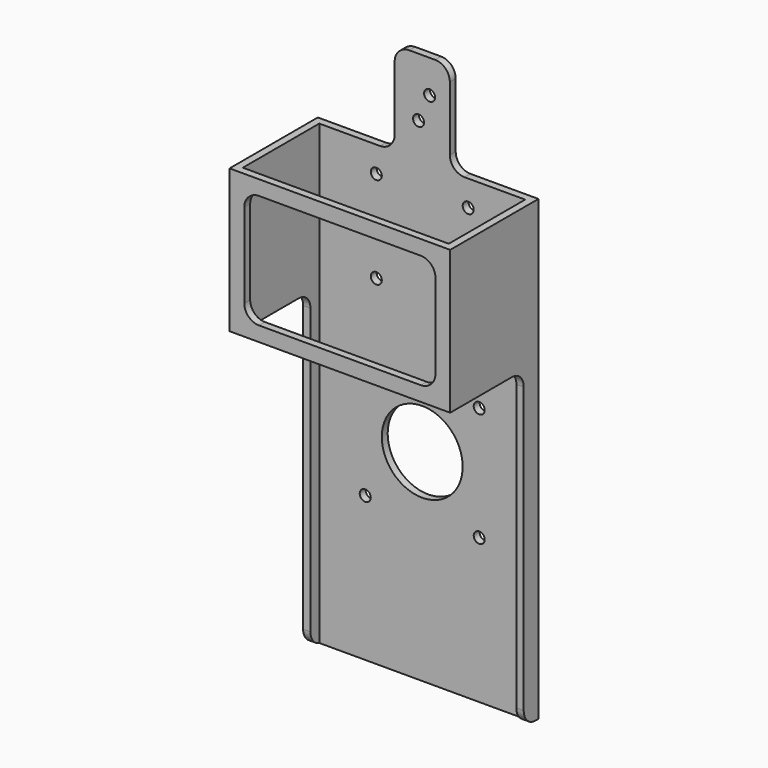
from build123d import *

# Parameters (mm, degrees)
F0_W      = 60
F0_H      = 30
F1_DEPTH  = 150
F2_T      = -2
F4_D      = 3
F3_R      = 11
F5_DEPTH  = 30.001
F6_D      = 3
F7_D      = 3
F8_W      = 52
F8_H      = 31
F8_R      = 1.5
F8_W_2    = 60
F8_H_2    = 85.5
F8_R_2    = 11
F8_W_3    = 15
F8_H_3    = 25.5
F8_W_4    = 22.5
F9_DEPTH  = 25
F10_DEPTH = 30.001
F11_F1_R  = 4
F11_F2_R  = 4
F11_F3_R  = 4
F11_F4_R  = 4
F11_F5_R  = 4
F11_F6_R  = 4
F11_F7_R  = 4
F11_F8_R  = 4
F11_F9_R  = 4
F11_F10_R = 4
F11_F11_R = 4


with BuildPart() as f1:
    # F0 (on Top) → F1 (new body)
    with BuildSketch(Plane.XY):
        Rectangle(F0_W, F0_H)
    extrude(amount=F1_DEPTH)

    # F2
    f2_openings = [f1.faces().sort_by_distance(p)[0] for p in [
        (0, 0, 150),
        (0, 0, 0),
    ]]
    offset(amount=F2_T, openings=f2_openings)

    # F4 (through all)
    with Locations(Plane(origin=(0, 15, 0), x_dir=(-1, 0, 0), z_dir=(0, 1, 0))):
        with Locations((-12.5, 117.5), (12.5, 117.5), (-12.5, 92.5), (12.5, 92.5)):
            Hole(F4_D / 2)

    # F3 (on face) → F5 (cut, through all)
    with BuildSketch(Plane(origin=(0, 15, 0), x_dir=(-1, 0, 0), z_dir=(0, 1, 0))):
        with Locations((0, 55)):
            Circle(F3_R)
    extrude(amount=-F5_DEPTH, mode=Mode.SUBTRACT)

    # F6 (through all)
    with Locations(Plane(origin=(0, 15, 0), x_dir=(-1, 0, 0), z_dir=(0, 1, 0))):
        with Locations((-15.5, 70.5), (15.5, 70.5), (-15.5, 39.5), (15.5, 39.5)):
            Hole(F6_D / 2)

    # F7 (through all)
    with Locations(Plane(origin=(0, 15, 0), x_dir=(-1, 0, 0), z_dir=(0, 1, 0))):
        with Locations((-2, 141), (1, 134)):
            Hole(F7_D / 2)

    # F8 (on face) → F9 (cut)
    with BuildSketch(Plane.XZ.offset(15)):
        with Locations((0, 105)):
            Rectangle(F8_W, F8_H)
        with Locations((-12.5, 92.5)):
            Circle(F8_R, mode=Mode.SUBTRACT)
        with Locations((-12.5, 117.5)):
            Circle(F8_R, mode=Mode.SUBTRACT)
        with Locations((12.5, 92.5)):
            Circle(F8_R, mode=Mode.SUBTRACT)
        with Locations((12.5, 117.5)):
            Circle(F8_R, mode=Mode.SUBTRACT)
        with Locations((0, 42.75)):
            Rectangle(F8_W_2, F8_H_2)
        with Locations((-15.5, 39.5)):
            Circle(F8_R, mode=Mode.SUBTRACT)
        with Locations((-15.5, 70.5)):
            Circle(F8_R, mode=Mode.SUBTRACT)
        with Locations((0, 55)):
            Circle(F8_R_2, mode=Mode.SUBTRACT)
        with Locations((15.5, 39.5)):
            Circle(F8_R, mode=Mode.SUBTRACT)
        with Locations((15.5, 70.5)):
            Circle(F8_R, mode=Mode.SUBTRACT)
        with Locations((0, 137.25)):
            Rectangle(F8_W_3, F8_H_3)
        with Locations((-1, 134)):
            Circle(F8_R, mode=Mode.SUBTRACT)
        with Locations((2, 141)):
            Circle(F8_R, mode=Mode.SUBTRACT)
        with Locations((18.75, 137.25)):
            Rectangle(F8_W_4, F8_H_3)
        with Locations((-18.75, 137.25)):
            Rectangle(F8_W_4, F8_H_3)
    extrude(amount=-F9_DEPTH, mode=Mode.SUBTRACT)

    # F8 (on face) → F10 (cut, through all)
    with BuildSketch(Plane.XZ.offset(15)):
        with Locations((-18.75, 137.25)):
            Rectangle(F8_W_4, F8_H_3)
        with Locations((18.75, 137.25)):
            Rectangle(F8_W_4, F8_H_3)
    extrude(amount=-F10_DEPTH, mode=Mode.SUBTRACT)

    # F11: fillet of radius 4 on 12 edges, made by hand

    # F11_f1
    f11_f1_edges = [f1.edges().sort_by_distance(p)[0] for p in [
        (29, 10, 0),
    ]]
    fillet(f11_f1_edges, radius=F11_F1_R)

    # F11_f2
    f11_f2_edges = [f1.edges().sort_by_distance(p)[0] for p in [
        (29, 10, 85.5),
    ]]
    fillet(f11_f2_edges, radius=F11_F2_R)

    # F11_f3
    f11_f3_edges = [f1.edges().sort_by_distance(p)[0] for p in [
        (7.5, 14, 124.5),
    ]]
    fillet(f11_f3_edges, radius=F11_F3_R)

    # F11_f4
    f11_f4_edges = [f1.edges().sort_by_distance(p)[0] for p in [
        (7.5, 14, 150),
    ]]
    fillet(f11_f4_edges, radius=F11_F4_R)

    # F11_f5
    f11_f5_edges = [f1.edges().sort_by_distance(p)[0] for p in [
        (-7.5, 14, 150),
    ]]
    fillet(f11_f5_edges, radius=F11_F5_R)

    # F11_f6
    f11_f6_edges = [f1.edges().sort_by_distance(p)[0] for p in [
        (-7.5, 14, 124.5),
    ]]
    fillet(f11_f6_edges, radius=F11_F6_R)

    # F11_f7
    f11_f7_edges = [f1.edges().sort_by_distance(p)[0] for p in [
        (-29, 10, 85.5),
    ]]
    fillet(f11_f7_edges, radius=F11_F7_R)

    # F11_f8
    f11_f8_edges = [f1.edges().sort_by_distance(p)[0] for p in [
        (26, -14, 89.5),
    ]]
    fillet(f11_f8_edges, radius=F11_F8_R)

    # F11_f9
    f11_f9_edges = [f1.edges().sort_by_distance(p)[0] for p in [
        (-26, -14, 89.5),
    ]]
    fillet(f11_f9_edges, radius=F11_F9_R)

    # F11_f10
    f11_f10_edges = [f1.edges().sort_by_distance(p)[0] for p in [
        (-26, -14, 120.5),
    ]]
    fillet(f11_f10_edges, radius=F11_F10_R)

    # F11_f11
    f11_f11_edges = [f1.edges().sort_by_distance(p)[0] for p in [
        (26, -14, 120.5),
    ]]
    fillet(f11_f11_edges, radius=F11_F11_R)


solid = f1.part
